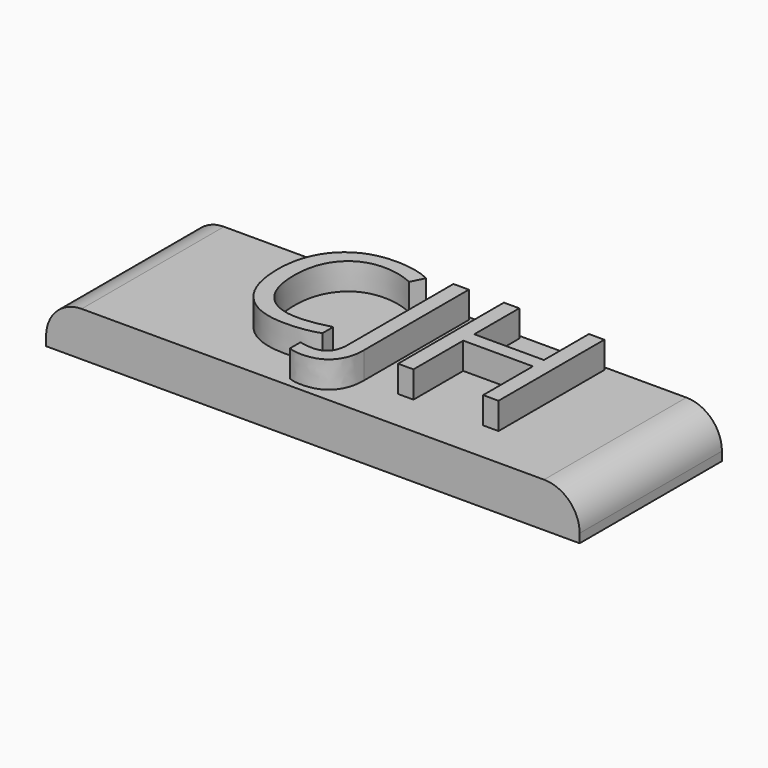
from build123d import *

# Parameters (mm, degrees)
F0_W         = 76.2
F0_H         = 25.4
F1_DEPTH     = 6.35
F2_TEXT_SIZE = 26.4583333333
F3_DEPTH     = 10.16
F4_R         = 5.08


# Not quite as in the source:
# - Text() gives the source's letters only with a copy of the font that has no kerning and outlines rounded to 1/6400 em; it was checked with that copy


with BuildPart() as f1:
    # F0 (on Top) → F1 (new body)
    with BuildSketch(Plane.XY):
        Rectangle(F0_W, F0_H)
    extrude(amount=F1_DEPTH)

    # F2 (on Top) → F3 (join)
    with BuildSketch(Plane.XY):
        with Locations((-18.9751426881, -6.7113825609)):
            Text('CJH', F2_TEXT_SIZE, font='Open Sans', text_align=(TextAlign.LEFT, TextAlign.BOTTOM))
    extrude(amount=F3_DEPTH)

    # F4
    f4_edges = [f1.edges().sort_by_distance(p)[0] for p in [
        (-38.1, 0, 6.35),
        (38.1, 0, 6.35),
    ]]
    fillet(f4_edges, radius=F4_R)


solid = f1.part
